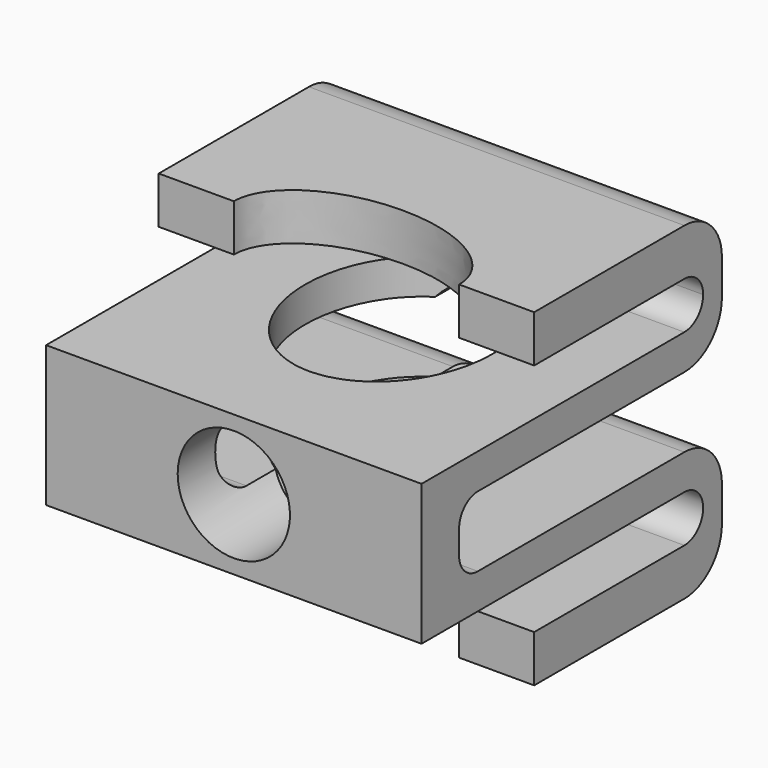
from build123d import *

# Parameters (mm, degrees)
F1_DEPTH      = 6.35
F4_D          = 3.7973
F6_DEPTH      = 2.38125
F6_DEPTH_BACK = 2.38125
F9_DEPTH      = 1.5875
F10_DEPTH     = 1.5875


with BuildPart() as f1:
    # F0 (on Right) → F1 (new body, symmetric)
    with BuildSketch(Plane.YZ):
        with BuildLine():
            Line((11.1125, 2.38125), (0, 2.38125))
            Line((0, 2.38125), (0, 0))
            Line((0, 0), (0, -2.38125))
            Line((0, -2.38125), (11.1125, -2.38125))
            ThreePointArc((11.1125, -2.38125), (11.673766, -2.613734), (11.90625, -3.175))
            ThreePointArc((11.90625, -3.175), (11.673766, -3.736266), (11.1125, -3.96875))
            Line((11.1125, -3.96875), (4.7625, -3.96875))
            Line((4.7625, -3.96875), (4.7625, -5.55625))
            Line((4.7625, -5.55625), (11.1125, -5.55625))
            ThreePointArc((11.1125, -5.55625), (12.235032, -5.091282), (12.7, -3.96875))
            Line((12.7, -3.96875), (12.7, -2.778125))
            ThreePointArc((12.7, -2.778125), (12.235032, -1.655593), (11.1125, -1.190625))
            Line((11.1125, -1.190625), (2.38125, -1.190625))
            ThreePointArc((2.38125, -1.190625), (1.819984, -0.958141), (1.5875, -0.396875))
            Line((1.5875, -0.396875), (1.5875, 0))
            Line((1.5875, 0), (1.5875, 0.396875))
            ThreePointArc((1.5875, 0.396875), (1.819984, 0.958141), (2.38125, 1.190625))
            Line((2.38125, 1.190625), (11.1125, 1.190625))
            ThreePointArc((11.1125, 1.190625), (12.235032, 1.655593), (12.7, 2.778125))
            Line((12.7, 2.778125), (12.7, 3.96875))
            ThreePointArc((12.7, 3.96875), (12.235032, 5.091282), (11.1125, 5.55625))
            Line((11.1125, 5.55625), (4.7625, 5.55625))
            Line((4.7625, 5.55625), (4.7625, 3.96875))
            Line((4.7625, 3.96875), (11.1125, 3.96875))
            ThreePointArc((11.1125, 3.96875), (11.673766, 3.736266), (11.90625, 3.175))
            ThreePointArc((11.90625, 3.175), (11.673766, 2.613734), (11.1125, 2.38125))
        make_face()
    extrude(amount=F1_DEPTH, both=True)

    # F4 (through all)
    with Locations(Plane.XZ):
        with Locations((0, 0)):
            Hole(F4_D / 2)

    # F5 (on face) → F6 (cut, two sides)
    with BuildSketch(Plane.XY) as f6_sk:
        with BuildLine():
            add(Edge.make_bspline(
                [(0, 10.795), (-5.499261, 10.795), (-2.749631, 5.08), (0, -0.635), (2.749631, 5.08), (5.499261, 10.795), (0, 10.795)],
                knots=[0, 0, 0, 2.094395, 2.094395, 4.18879, 4.18879, 6.283185, 6.283185, 6.283185], degree=2, weights=[1, 0.5, 1, 0.5, 1, 0.5, 1]))
        make_face()
    extrude(amount=-F6_DEPTH, mode=Mode.SUBTRACT)
    extrude(f6_sk.sketch, amount=F6_DEPTH_BACK, mode=Mode.SUBTRACT)

    # F7 (on face) → F9 (cut, through all)
    with BuildSketch(Plane.XY.offset(5.55625)):
        with BuildLine():
            Line((-3.81, 4.7625), (3.81, 4.7625))
            add(Edge.make_bspline(
                [(3.81, 4.7625), (3.81, 7.14375), (0, 7.14375), (-3.81, 7.14375), (-3.81, 4.7625)],
                knots=[0, 0, 0, 1.570796, 1.570796, 3.141593, 3.141593, 3.141593], degree=2, weights=[1, 0.707107, 1, 0.707107, 1]))
        make_face()
    extrude(amount=-F9_DEPTH, mode=Mode.SUBTRACT)

    # F8 (on face) → F10 (cut, through all)
    with BuildSketch(Plane(origin=(0, 0, -5.55625), x_dir=(1, 0, 0), z_dir=(0, 0, -1))):
        with BuildLine():
            Line((3.81, -4.7625), (-3.81, -4.7625))
            add(Edge.make_bspline(
                [(-3.81, -4.7625), (-3.81, -7.14375), (0, -7.14375), (3.81, -7.14375), (3.81, -4.7625)],
                knots=[0, 0, 0, 1.570796, 1.570796, 3.141593, 3.141593, 3.141593], degree=2, weights=[1, 0.707107, 1, 0.707107, 1]))
        make_face()
    extrude(amount=-F10_DEPTH, mode=Mode.SUBTRACT)


solid = f1.part
